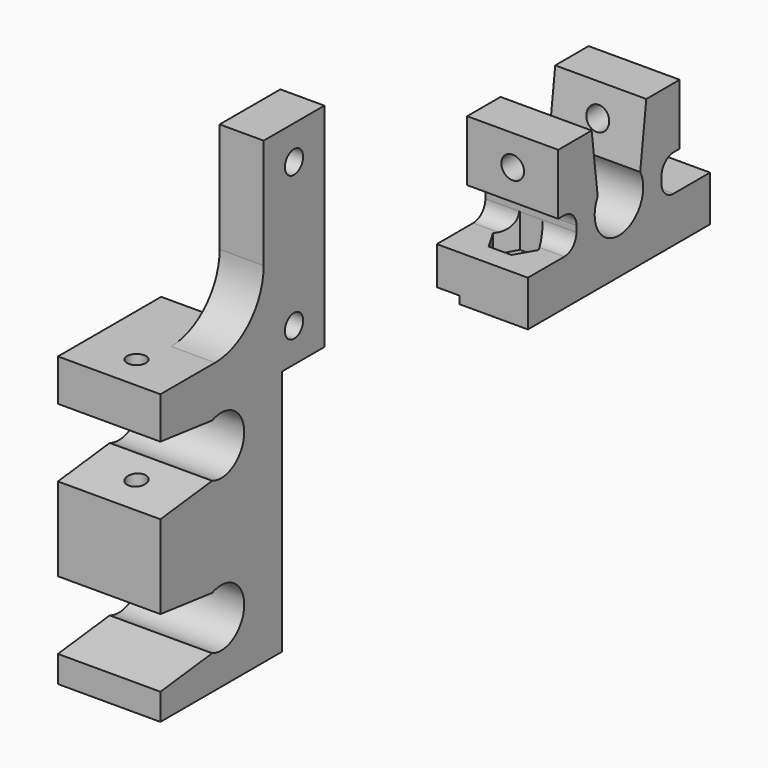
from build123d import *

# Parameters (mm, degrees)
F0_R           = 3.8
F0_R_2         = 1.5
F1_DEPTH       = 3.5
F3_DEPTH       = 2.3
F4_DEPTH       = 10
F6_DEPTH       = 13.501
F7_R           = 1.25
F8_DEPTH       = 30
F9_R           = 4
F10_DEPTH      = 12
F11_R          = 2
F12_R          = 1.5
F13_DEPTH      = 34.001
F13_DEPTH_BACK = 3
F14_DEPTH      = 2.5
F14_DEPTH_BACK = 2
F16_DEPTH      = 22.001
F17_R          = 1.5
F18_DEPTH      = 74.8861283789
F19_DEPTH      = 2.5
F20_R          = 2
F21_W          = 3
F21_H          = 30
F22_DEPTH      = 1


with BuildPart() as f1:
    # F0 (on Right) → F1 (new body)
    with BuildSketch(Plane.YZ):
        with BuildLine():
            Line((17, 32.5), (7, 32.5))
            Line((7, 32.5), (7, 18))
            ThreePointArc((7, 18), (4.6568542495, 12.3431457505), (-1, 10))
            Line((-1, 10), (-10, 10))
            Line((-10, 10), (-10, -28))
            Line((-10, -28), (10, -28))
            Line((10, -28), (10, 4.5))
            Line((10, 4.5), (17, 4.5))
            Line((17, 4.5), (17, 32.5))
        make_face()
        with Locations((0, -20)):
            Circle(F0_R, mode=Mode.SUBTRACT)
        Circle(F0_R, mode=Mode.SUBTRACT)
        with Locations((12, 9)):
            Circle(F0_R_2, mode=Mode.SUBTRACT)
        with Locations((12, 28)):
            Circle(F0_R_2, mode=Mode.SUBTRACT)
    extrude(amount=F1_DEPTH)

    # F2 (on face) → F3 (join)
    with BuildSketch(Plane(origin=(0, 0, 0), x_dir=(0, -1, 0), z_dir=(-1, 0, 0))):
        with BuildLine():
            Line((-17, 4.5), (-10, 4.5))
            Line((-10, 4.5), (-7, 10))
            Line((-7, 10), (1, 10))
            ThreePointArc((1, 10), (-4.6568542495, 12.3431457505), (-7, 18))
            Line((-7, 18), (-7, 32.5))
            Line((-7, 32.5), (-17, 32.5))
            Line((-17, 32.5), (-17, 4.5))
        make_face()
        Polygon((-10.479440264, 11.7876928494), (-8.8255073065, 9.0770030653), (-10.3460670425, 6.2893102159), (-13.520559736, 6.2123071506), (-15.1744926935, 8.9229969347), (-13.6539329575, 11.7106897841), align=None, mode=Mode.SUBTRACT)
        Polygon((-12, 31.1754264805), (-9.25, 29.5877132403), (-9.25, 26.4122867597), (-12, 24.8245735195), (-14.75, 26.4122867597), (-14.75, 29.5877132403), align=None, mode=Mode.SUBTRACT)
    extrude(amount=F3_DEPTH)

    # F4 (add): a face of the model
    f4_faces = [f1.faces().sort_by_distance(p)[0] for p in [
        (0, -0.112326268, -9.0769957675),
    ]]
    extrude(f4_faces, amount=F4_DEPTH)

    # F5 (on face) → F6 (cut, through all)
    with BuildSketch(Plane.YZ.offset(3.5)):
        with BuildLine():
            ThreePointArc((-1.4798648587, -3.5), (2.0995849039, -3.1672927291), (3.8, 0))
            ThreePointArc((3.8, 0), (2.0995849039, 3.1672927291), (-1.4798648587, 3.5))
            Line((-1.4798648587, 3.5), (-1.4798648587, -3.5))
        make_face()
        with BuildLine():
            Line((-1.4798648587, -3.5), (-1.4798648587, 3.5))
            ThreePointArc((-1.4798648587, 3.5), (-3.8, 0), (-1.4798648587, -3.5))
        make_face()
        with BuildLine():
            ThreePointArc((-1.4798648587, -3.5), (-3.8, 0), (-1.4798648587, 3.5))
            Line((-1.4798648587, 3.5), (-10, 4.5))
            Line((-10, 4.5), (-10, -4.5))
            Line((-10, -4.5), (-1.4798648587, -3.5))
        make_face()
        with BuildLine():
            ThreePointArc((-1.4798648587, -23.5), (2.0995849039, -23.1672927291), (3.8, -20))
            ThreePointArc((3.8, -20), (2.0995849039, -16.8327072709), (-1.4798648587, -16.5))
            Line((-1.4798648587, -16.5), (-1.4798648587, -23.5))
        make_face()
        with BuildLine():
            Line((-1.4798648587, -23.5), (-1.4798648587, -16.5))
            ThreePointArc((-1.4798648587, -16.5), (-3.8, -20), (-1.4798648587, -23.5))
        make_face()
        with BuildLine():
            ThreePointArc((-1.4798648587, -23.5), (-3.8, -20), (-1.4798648587, -16.5))
            Line((-1.4798648587, -16.5), (-10, -15.5))
            Line((-10, -15.5), (-10, -24.5))
            Line((-10, -24.5), (-1.4798648587, -23.5))
        make_face()
    extrude(amount=-F6_DEPTH, mode=Mode.SUBTRACT)

    # F7 (on face) → F8 (cut)
    with BuildSketch(Plane.XY.offset(10)):
        with Locations((-3.25, -5.5)):
            Circle(F7_R)
    extrude(amount=-F8_DEPTH, mode=Mode.SUBTRACT)


with BuildPart() as f10:
    # F9 (on Right) → F10 (new body)
    with BuildSketch(Plane.YZ):
        Polygon((39.8851283789, 0), (69.8851283789, 0), (69.8851283789, 6), (61.8851283789, 6), (61.8851283789, 10.8), (64.8851283789, 10.8), (64.8851283789, 18.8), (44.8851283789, 18.8), (44.8851283789, 10.8), (47.8851283789, 10.8), (47.8851283789, 6), (39.8851283789, 6), align=None)
        with Locations((54.8851283789, 8.8)):
            Circle(F9_R, mode=Mode.SUBTRACT)
    extrude(amount=F10_DEPTH)

    # F11
    f11_edges = [f10.edges().sort_by_distance(p)[0] for p in [
        (6, 47.885128, 6),
        (6, 61.885128, 6),
    ]]
    fillet(f11_edges, radius=F11_R)

    # F12 (on face) → F13 (cut, two sides)
    with BuildSketch(Plane.XY.offset(6)) as f13_sk:
        with BuildLine():
            Line((4.5857864376, 45.8851283789), (7.4142135624, 45.8851283789))
            ThreePointArc((7.4142135624, 45.8851283789), (6, 46.8851283789), (4.5857864376, 45.8851283789))
        make_face()
        with BuildLine():
            ThreePointArc((4.5857864376, 45.8851283789), (5.7463470319, 43.9067305394), (7.5, 45.3851283789))
            ThreePointArc((7.5, 45.3851283789), (7.4783978395, 45.638781347), (7.4142135624, 45.8851283789))
            Line((7.4142135624, 45.8851283789), (4.5857864376, 45.8851283789))
        make_face()
        with Locations((6, 64.3851283789)):
            Circle(F12_R)
    extrude(amount=-F13_DEPTH, mode=Mode.SUBTRACT)
    extrude(f13_sk.sketch, amount=F13_DEPTH_BACK, mode=Mode.SUBTRACT)

    # F12 (on face) → F14 (cut, two sides)
    with BuildSketch(Plane.XY.offset(6)) as f14_sk:
        Polygon((7.5067365177, 42.7883845718), (9.0022143629, 45.3916285765), (7.4954778452, 47.9883723835), (4.4932634823, 47.9818721859), (2.9977856371, 45.3786281813), (4.5045221548, 42.7818843742), align=None)
        with Locations((6, 45.3851283789)):
            Circle(F12_R, mode=Mode.SUBTRACT)
        Polygon((4.5045221548, 66.9883723835), (2.9977856371, 64.3916285765), (4.4932634823, 61.7883845718), (7.4954778452, 61.7818843742), (9.0022143629, 64.3786281813), (7.5067365177, 66.9818721859), align=None)
        with Locations((6, 64.3851283789)):
            Circle(F12_R, mode=Mode.SUBTRACT)
    extrude(amount=-F14_DEPTH, mode=Mode.SUBTRACT)
    extrude(f14_sk.sketch, amount=F14_DEPTH_BACK, mode=Mode.SUBTRACT)

    # F15 (on face) → F16 (cut, through all)
    with BuildSketch(Plane.YZ.offset(12)):
        with BuildLine():
            ThreePointArc((51.3851283789, 10.7364916731), (54.8851283789, 12.8), (58.3851283789, 10.7364916731))
            Line((58.3851283789, 10.7364916731), (59.3851283789, 18.8))
            Line((59.3851283789, 18.8), (50.3851283789, 18.8))
            Line((50.3851283789, 18.8), (51.3851283789, 10.7364916731))
        make_face()
    extrude(amount=-F16_DEPTH, mode=Mode.SUBTRACT)

    # F17 (on face) → F18 (cut, through all)
    with BuildSketch(Plane(origin=(0, 64.8851283789, 0), x_dir=(-1, 0, 0), z_dir=(0, 1, 0))):
        with Locations((-6, 14.8)):
            Circle(F17_R)
    extrude(amount=-F18_DEPTH, mode=Mode.SUBTRACT)

    # F17 (on face) → F19 (cut)
    with BuildSketch(Plane(origin=(0, 64.8851283789, 0), x_dir=(-1, 0, 0), z_dir=(0, 1, 0))):
        Polygon((-4.4988893001, 17.4), (-7.5011106999, 17.4), (-9.0022213998, 14.8), (-7.5011106999, 12.2), (-4.4988893001, 12.2), (-2.9977786002, 14.8), align=None)
        with Locations((-6, 14.8)):
            Circle(F17_R, mode=Mode.SUBTRACT)
    extrude(amount=-F19_DEPTH, mode=Mode.SUBTRACT)

    # F20
    f20_edges = [f10.edges().sort_by_distance(p)[0] for p in [
        (6, 61.885128, 10.8),
        (6, 47.885128, 10.8),
    ]]
    fillet(f20_edges, radius=F20_R)

    # F21 (on face) → F22 (cut)
    with BuildSketch(Plane(origin=(0, 0, 0), x_dir=(1, 0, 0), z_dir=(0, 0, -1))):
        with Locations((1.5, -54.8851283789)):
            Rectangle(F21_W, F21_H)
    extrude(amount=-F22_DEPTH, mode=Mode.SUBTRACT)


solid = Compound([f1.part, f10.part])
